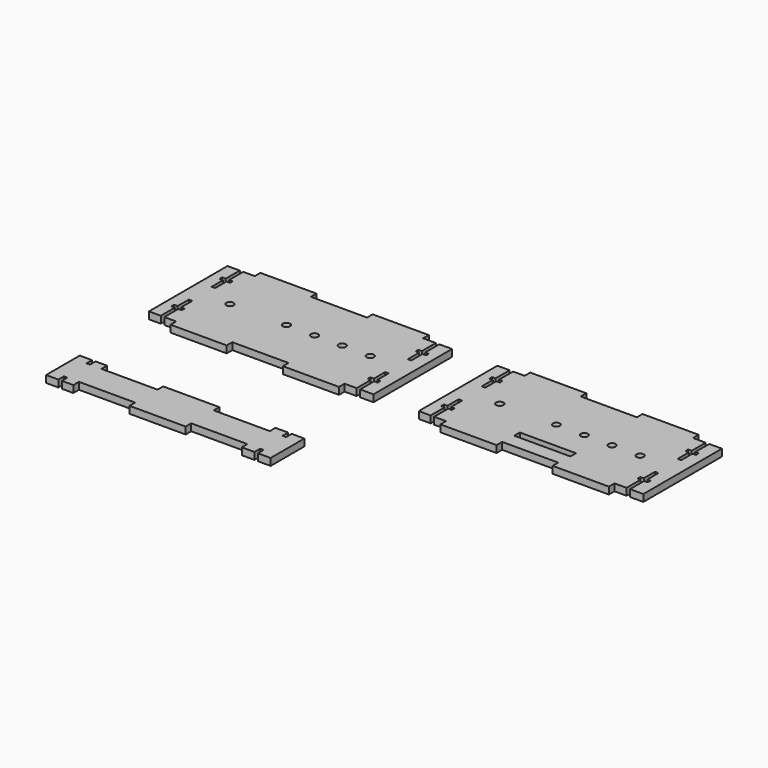
from build123d import *

# Parameters (mm, degrees)
F0_W     = 25.4
F0_H     = 3.175
F0_R     = 1.651
F0_R_2   = 1.5875
F1_DEPTH = 3.175


# Not quite as in the source:
# - a length typed as a fraction of an inch, garbled in the dataset ("3 / 203.2 mm" for 3/8 in), is restored


with BuildPart() as f1:
    # F0 (on Top) → F1 (new body)
    with BuildSketch(Plane.XY):
        Polygon((14.6100838328, -22.482711039), (19.9830344046, -22.482711039), (19.9830344046, -25.657711039), (45.3830344046, -25.657711039), (45.3830344046, -22.482711039), (70.7830344046, -22.482711039), (70.7830344046, -25.657711039), (96.1830344046, -25.657711039), (96.1830344046, -22.482711039), (101.6479595924, -22.482711039), (101.6479595924, -14.545211039), (100.2515068019, -14.545211039), (100.2515068019, -12.957711039), (101.8390068019, -12.957711039), (101.8390068019, -6.607711039), (103.4265068019, -6.607711039), (103.4265068019, -12.957711039), (104.8229595924, -12.957711039), (104.8229595924, -14.545211039), (103.2354595924, -14.545211039), (103.2354595924, -22.482711039), (109.2496332611, -22.482711039), (109.2496332611, 21.967288961), (103.5178316141, 21.967288961), (103.5178316141, 14.029788961), (105.1053316141, 14.029788961), (105.1053316141, 12.442288961), (103.5178316141, 12.442288961), (103.5178316141, 6.092288961), (101.9303316141, 6.092288961), (101.9303316141, 12.442288961), (100.3428316141, 12.442288961), (100.3428316141, 14.029788961), (101.9303316141, 14.029788961), (101.9303316141, 21.967288961), (96.1830344046, 21.967288961), (96.1830344046, 25.142288961), (70.7830344046, 25.142288961), (70.7830344046, 21.967288961), (45.3830344046, 21.967288961), (45.3830344046, 25.142288961), (19.9830344046, 25.142288961), (19.9830344046, 21.967288961), (14.7933832611, 21.967288961), (14.7933832611, 14.029788961), (16.3808832611, 14.029788961), (16.3808832611, 12.442288961), (14.7933832611, 12.442288961), (14.7933832611, 6.092288961), (13.2058832611, 6.092288961), (13.2058832611, 12.442288961), (11.6183832611, 12.442288961), (11.6183832611, 14.029788961), (13.2058832611, 14.029788961), (13.2058832611, 21.967288961), (7.6496332611, 21.967288961), (7.6496332611, -22.482711039), (13.0225838328, -22.482711039), (13.0225838328, -14.545211039), (11.4350838328, -14.545211039), (11.4350838328, -12.957711039), (13.0225838328, -12.957711039), (13.0225838328, -6.607711039), (13.8163338328, -6.607711039), (14.6100838328, -6.607711039), (14.6100838328, -12.957711039), (16.1975838328, -12.957711039), (16.1975838328, -14.545211039), (14.6100838328, -14.545211039), align=None)
        with Locations((58.4496332611, -14.545211039)):
            Rectangle(F0_W, F0_H, mode=Mode.SUBTRACT)
        with Locations((26.5240816141, -0.257711039)):
            Circle(F0_R, mode=Mode.SUBTRACT)
        with Locations((52.0996332611, -0.257711039)):
            Circle(F0_R_2, mode=Mode.SUBTRACT)
        with Locations((64.7996332611, -0.257711039)):
            Circle(F0_R_2, mode=Mode.SUBTRACT)
        with Locations((77.3240816141, -0.257711039)):
            Circle(F0_R, mode=Mode.SUBTRACT)
        with Locations((90.0240816141, -0.257711039)):
            Circle(F0_R, mode=Mode.SUBTRACT)
    extrude(amount=F1_DEPTH)


with BuildPart() as f1b:
    # F0 (on Top) → F1, piece 2 (new body)
    with BuildSketch(Plane.XY):
        Polygon((-107.4923401093, -22.482711039), (-102.1193895375, -22.482711039), (-102.1193895375, -25.657711039), (-76.7193895375, -25.657711039), (-76.7193895375, -22.482711039), (-51.3193895375, -22.482711039), (-51.3193895375, -25.657711039), (-25.9193895375, -25.657711039), (-25.9193895375, -22.482711039), (-20.4544643497, -22.482711039), (-20.4544643497, -14.545211039), (-21.8509171402, -14.545211039), (-21.8509171402, -12.957711039), (-20.2634171402, -12.957711039), (-20.2634171402, -6.607711039), (-18.6759171402, -6.607711039), (-18.6759171402, -12.957711039), (-17.2794643497, -12.957711039), (-17.2794643497, -14.545211039), (-18.8669643497, -14.545211039), (-18.8669643497, -22.482711039), (-12.852790681, -22.482711039), (-12.852790681, 21.967288961), (-18.584592328, 21.967288961), (-18.584592328, 14.029788961), (-16.997092328, 14.029788961), (-16.997092328, 12.442288961), (-18.584592328, 12.442288961), (-18.584592328, 6.092288961), (-20.172092328, 6.092288961), (-20.172092328, 12.442288961), (-21.759592328, 12.442288961), (-21.759592328, 14.029788961), (-20.172092328, 14.029788961), (-20.172092328, 21.967288961), (-25.9193895375, 21.967288961), (-25.9193895375, 25.142288961), (-51.3193895375, 25.142288961), (-51.3193895375, 21.967288961), (-76.7193895375, 21.967288961), (-76.7193895375, 25.142288961), (-102.1193895375, 25.142288961), (-102.1193895375, 21.967288961), (-107.309040681, 21.967288961), (-107.309040681, 14.029788961), (-105.721540681, 14.029788961), (-105.721540681, 12.442288961), (-107.309040681, 12.442288961), (-107.309040681, 6.092288961), (-108.896540681, 6.092288961), (-108.896540681, 12.442288961), (-110.484040681, 12.442288961), (-110.484040681, 14.029788961), (-108.896540681, 14.029788961), (-108.896540681, 21.967288961), (-114.452790681, 21.967288961), (-114.452790681, -22.482711039), (-109.0798401093, -22.482711039), (-109.0798401093, -14.545211039), (-110.6673401093, -14.545211039), (-110.6673401093, -12.957711039), (-109.0798401093, -12.957711039), (-109.0798401093, -6.607711039), (-108.2860901093, -6.607711039), (-107.4923401093, -6.607711039), (-107.4923401093, -12.957711039), (-105.9048401093, -12.957711039), (-105.9048401093, -14.545211039), (-107.4923401093, -14.545211039), align=None)
        with Locations((-95.578342328, -0.257711039)):
            Circle(F0_R, mode=Mode.SUBTRACT)
        with Locations((-69.9939727783, -0.257711039)):
            Circle(F0_R, mode=Mode.SUBTRACT)
        with Locations((-57.2999119759, -0.257711039)):
            Circle(F0_R, mode=Mode.SUBTRACT)
        with Locations((-44.778342328, -0.257711039)):
            Circle(F0_R, mode=Mode.SUBTRACT)
        with Locations((-32.078342328, -0.257711039)):
            Circle(F0_R, mode=Mode.SUBTRACT)
    extrude(amount=F1_DEPTH)


with BuildPart() as f1c:
    # F0 (on Top) → F1, piece 3 (new body)
    with BuildSketch(Plane.XY):
        Polygon((-100.0680774225, -80.0153038105), (-74.6680774225, -80.0153038105), (-74.6680774225, -83.1903038105), (-49.2680774225, -83.1903038105), (-49.2680774225, -80.0153038105), (-23.8680774225, -80.0153038105), (-23.8680774225, -83.1903038105), (-18.120780213, -83.1903038105), (-18.120780213, -80.0231885267), (-16.533280213, -80.0231885267), (-16.533280213, -83.1903038105), (-10.8014785661, -83.1903038105), (-10.8014785661, -64.1403038105), (-16.533280213, -64.1403038105), (-16.533280213, -67.3043401082), (-18.120780213, -67.3043401082), (-18.120780213, -64.1403038105), (-23.8680774225, -64.1403038105), (-23.8680774225, -67.3153038105), (-49.2680774225, -67.3153038105), (-49.2680774225, -64.1403038105), (-74.6680774225, -64.1403038105), (-74.6680774225, -67.3153038105), (-100.0680774225, -67.3153038105), (-100.0680774225, -64.1403038105), (-105.2577285661, -64.1403038105), (-105.2577285661, -67.3043401082), (-106.8452285661, -67.3043401082), (-106.8452285661, -64.1403038105), (-112.4014785661, -64.1403038105), (-112.4014785661, -83.1903038105), (-106.8452285661, -83.1903038105), (-106.8452285661, -80.0153038105), (-105.2577285661, -80.0153038105), (-105.2577285661, -83.1903038105), (-100.0680774225, -83.1903038105), align=None)
    extrude(amount=F1_DEPTH)


solid = Compound([f1.part, f1b.part, f1c.part])
